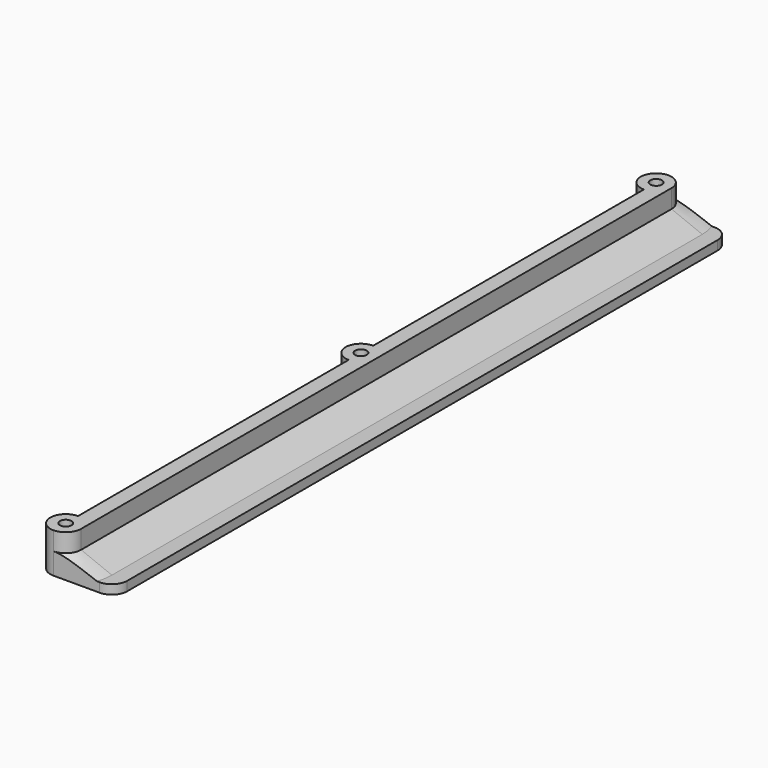
from build123d import *

# Parameters (mm, degrees)
F1_DEPTH       = 250
F3_D           = 3.7973
F3_CSINK_D     = 7.7978
F3_CSINK_ANGLE = 82
F2_W           = 5
F2_H           = 110
F4_DEPTH       = 13.001
F5_R           = 4.99999
F6_T1_DEPTH    = 240.00002
F6_T6_ANGLE    = 359.64
F6_T12_ANGLE   = 359.64


# Not quite as in the source:
# - a fillet or chamfer that OpenCascade refuses, or shapes differently, is made with other operations: its cross-section is extruded or revolved along the edge and cut away or added
# - a fillet or chamfer is up to 0.001 mm smaller than in the source, because OpenCascade refuses the exact size


with BuildPart() as f1:
    # F0 (on Front) → F1 (new body)
    with BuildSketch(Plane.XZ):
        Polygon((-15, 13), (-25, 13), (-25, 0), (0, 0), (0, 3), (-15, 3), align=None)
    extrude(amount=F1_DEPTH)

    # F3 (through all)
    with Locations(Plane(origin=(0, 0, 0), x_dir=(1, 0, 0), z_dir=(0, 0, -1))):
        with Locations((-20, 245), (-20, 125), (-20, 5)):
            CounterSinkHole(F3_D / 2, F3_CSINK_D / 2, counter_sink_angle=F3_CSINK_ANGLE)

    # F2 (on face) → F4 (cut, through all)
    with BuildSketch(Plane(origin=(0, 0, 0), x_dir=(1, 0, 0), z_dir=(0, 0, -1))):
        with Locations((-22.5, 185)):
            Rectangle(F2_W, F2_H)
        with Locations((-22.5, 65)):
            Rectangle(F2_W, F2_H)
    extrude(amount=-F4_DEPTH, mode=Mode.SUBTRACT)

    # F5 (radius 5 in the source; OpenCascade refuses exactly that, so slightly less here)
    f5_edges = [f1.edges().sort_by_distance(p)[0] for p in [
        (-25, 0, 6.5),
        (-25, -10, 6.5),
        (-25, -120, 6.5),
        (-25, -130, 6.5),
        (-25, -240, 6.5),
        (-25, -250, 6.5),
        (-15, -250, 8),
        (0, -250, 1.5),
        (-15, 0, 8),
        (0, 0, 1.5),
    ]]
    fillet(f5_edges, radius=F5_R)

    # F6: chamfer of 4 x 10 on 1 edges, made by hand

    # F6_s2 → F6_t1 (join)
    with BuildSketch(Plane.XZ.offset(4.99999)):
        Polygon((-15, 7), (-5, 3), (-15, 3), align=None)
    extrude(amount=F6_T1_DEPTH)


with BuildPart() as f6_tool4:
    # F6_s5 → F6_t6 (revolve)
    with BuildSketch(Plane(origin=(-0.0322045944, -5.1254529469, 0), x_dir=(0, 0, 1), z_dir=(0.006283144, 0.9999802609, 0))):
        Polygon((7, -14.9681895603), (3, -4.9681895603), (3, -14.9681895603), align=None)
    revolve(axis=Axis((-19.99999, -4.99999, 3), (0, 0, -1)), revolution_arc=F6_T6_ANGLE)

    split(bisect_by=Plane.XZ, keep=Keep.TOP)

    split(bisect_by=Plane.YZ.offset(-20), keep=Keep.TOP)


with BuildPart() as f1_1:
    add(f1.part)

    # F6_t3: union F6_tool4
    add(f6_tool4.part)


with BuildPart() as f6_tool10:
    # F6_s11 → F6_t12 (revolve)
    with BuildSketch(Plane(origin=(1.538550391, -244.8646775786, 0), x_dir=(0, 0, 1), z_dir=(0.006283144, -0.9999802609, 0))):
        Polygon((7, 16.5389755517), (3, 6.5389755517), (3, 16.5389755517), align=None)
    revolve(axis=Axis((-19.99999, -245.00001, 3), (0, 0, 1)), revolution_arc=F6_T12_ANGLE)

    split(bisect_by=Plane.XZ.offset(250), keep=Keep.BOTTOM)

    split(bisect_by=Plane.YZ.offset(-20), keep=Keep.TOP)


with BuildPart() as f1_2:
    add(f1_1.part)

    # F6_t9: union F6_tool10
    add(f6_tool10.part)


solid = f1_2.part
